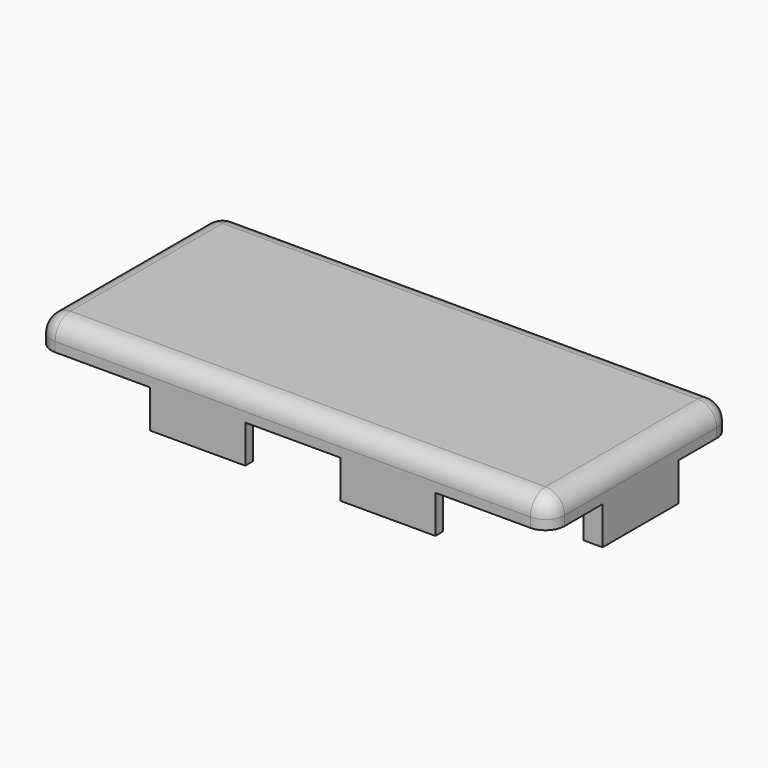
from build123d import *

# Parameters (mm, degrees)
F1_DEPTH = 1.5
F2_R     = 1
F3_W     = 24
F3_H     = 11
F4_DEPTH = 1
F5_R     = 0.99999
F6_W     = 2
F6_H     = 5
F6_W_2   = 1
F6_W_3   = 5
F6_H_2   = 0.5
F7_DEPTH = 2


# Not quite as in the source:
# - a fillet or chamfer is up to 0.001 mm smaller than in the source, because OpenCascade refuses the exact size


with BuildPart() as f1:
    # F0 (on Top) → F1 (new body)
    with BuildSketch(Plane.XY):
        with BuildLine():
            ThreePointArc((0, 1), (0.2928932188, 0.2928932188), (1, 0))
            Line((1, 0), (26, 0))
            ThreePointArc((26, 0), (26.7071067812, 0.2928932188), (27, 1))
            Line((27, 1), (27, 11))
            ThreePointArc((27, 11), (26.7071067812, 11.7071067812), (26, 12))
            Line((26, 12), (1, 12))
            ThreePointArc((1, 12), (0.2928932188, 11.7071067812), (0, 11))
            Line((0, 11), (0, 1))
        make_face()
    extrude(amount=F1_DEPTH)

    # F2
    f2_edges = [f1.edges().sort_by_distance(p)[0] for p in [
        (0, 6, 1.5),
        (0.292893, 0.292893, 1.5),
        (13.5, 0, 1.5),
        (26.707107, 0.292893, 1.5),
        (27, 6, 1.5),
        (26.707107, 11.707107, 1.5),
        (13.5, 12, 1.5),
        (0.292893, 11.707107, 1.5),
    ]]
    fillet(f2_edges, radius=F2_R)

    # F3 (on Top) → F4 (cut)
    with BuildSketch(Plane.XY):
        with Locations((14, 6)):
            Rectangle(F3_W, F3_H)
    extrude(amount=F4_DEPTH, mode=Mode.SUBTRACT)

    # F5 (radius 1 in the source; OpenCascade refuses exactly that, so slightly less here)
    f5_edges = [f1.edges().sort_by_distance(p)[0] for p in [
        (14, 11.5, 1),
        (2, 6, 1),
        (14, 0.5, 1),
        (26, 6, 1),
    ]]
    fillet(f5_edges, radius=F5_R)

    # F6 (on face) → F7 (join)
    with BuildSketch(Plane(origin=(0, 0, 0), x_dir=(1, 0, 0), z_dir=(0, 0, -1))):
        with Locations((1, -6)):
            Rectangle(F6_W, F6_H)
        with Locations((26.5, -6)):
            Rectangle(F6_W_2, F6_H)
        with Locations((8.5, -0.25)):
            Rectangle(F6_W_3, F6_H_2)
        with Locations((18.5, -0.25)):
            Rectangle(F6_W_3, F6_H_2)
        with Locations((18.5, -11.75)):
            Rectangle(F6_W_3, F6_H_2)
    extrude(amount=F7_DEPTH)


solid = f1.part
